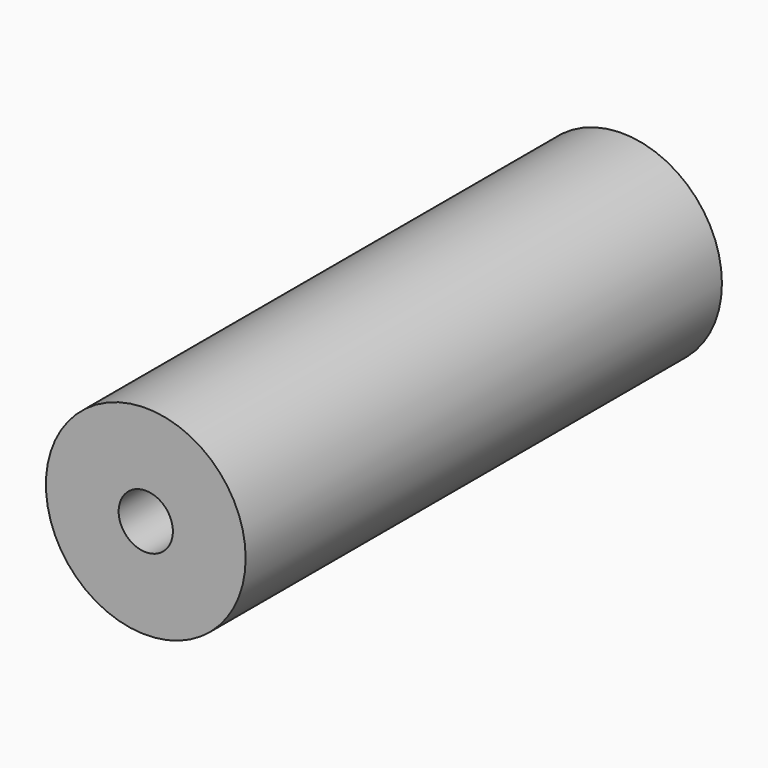
from build123d import *

# Parameters (mm, degrees)
F0_W = 11
F0_H = 10


# Not quite as in the source:
# - a feature names something its author has since deleted; it is built from what else it names


with BuildPart() as f1:
    # F0 (on Top) → F1 (revolve)
    with BuildSketch(Plane.XY):
        with Locations((9.45, 15)):
            Rectangle(F0_W, F0_H)
        with Locations((9.45, 25)):
            Rectangle(F0_W, F0_H)
        with Locations((9.45, 35)):
            Rectangle(F0_W, F0_H)
        Polygon((-0.15, 40), (3.95, 40), (14.95, 40), (14.95, 100), (-0.15, 100), align=None)
    revolve(axis=Axis((-0.15, 70, 0), (0, 1, 0)))


solid = f1.part
